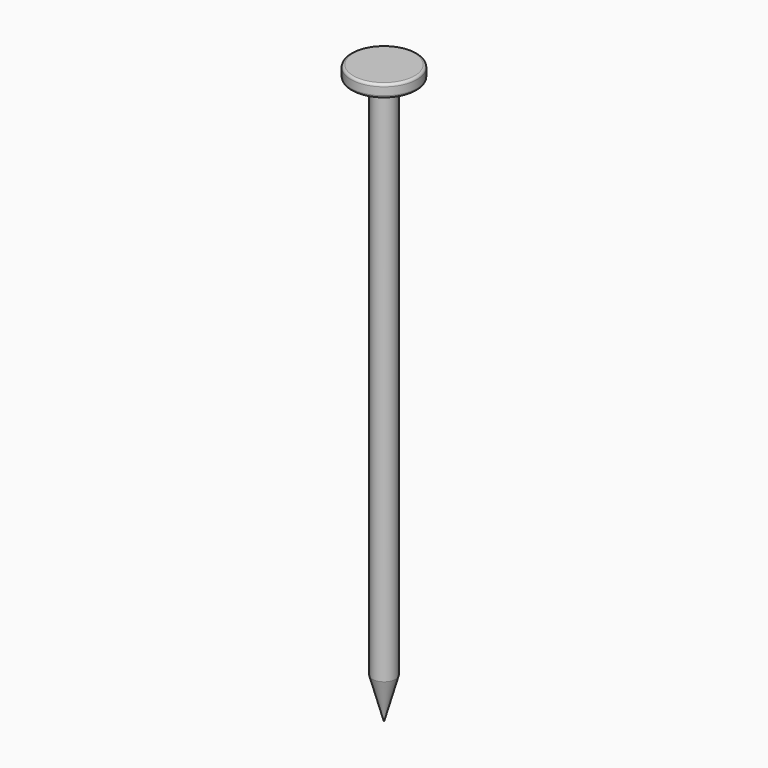
from build123d import *

# Parameters (mm, degrees)
F2_R = 1
F3_R = 0.3


# Not quite as in the source:
# - a feature names something its author has since deleted; it is built from what else it names


with BuildPart() as f1:
    # F0 (on Front) → F1 (revolve)
    with BuildSketch(Plane.XZ):
        Polygon((0, -70), (0, 0), (-1.4, 0), (-1.4, -1.6894261353), (-1.4, -65), align=None)
        Polygon((-1.4, -1.6894261353), (-1.4, 0), (-4, 0), (-4, -1.5247049741), align=None)
    revolve(axis=Axis((0, 0, -35), (0, 0, -1)))

    # F2
    f2_edges = [f1.edges().sort_by_distance(p)[0] for p in [
        (1.4, 0, -1.689426),
    ]]
    fillet(f2_edges, radius=F2_R)

    # F3
    f3_edges = [f1.edges().sort_by_distance(p)[0] for p in [
        (4, 0, 0),
        (4, 0, -1.524705),
    ]]
    fillet(f3_edges, radius=F3_R)


solid = f1.part
